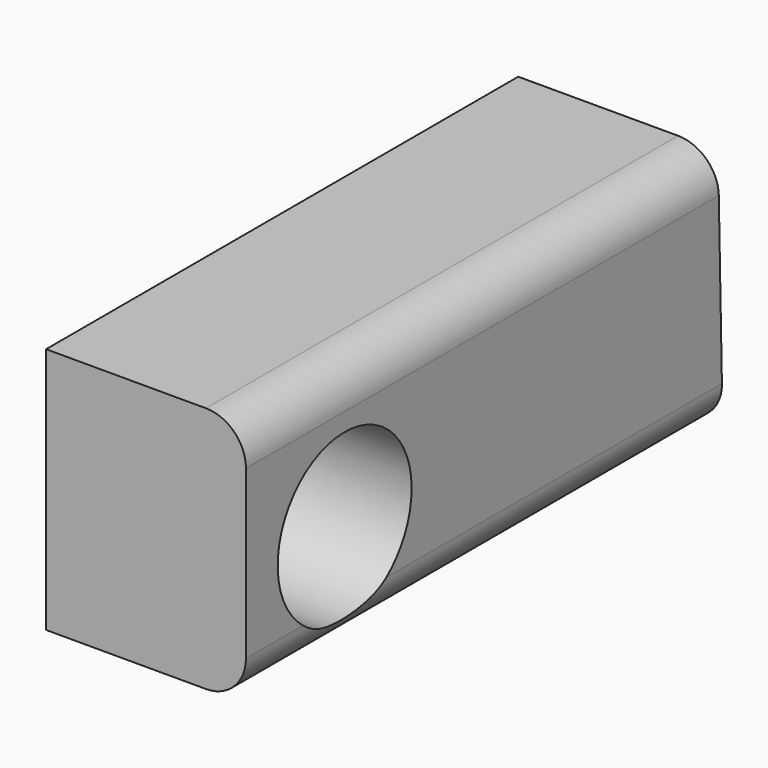
from build123d import *

# Parameters (mm, degrees)
F1_R        = 10.6370455912
F2_DEPTH    = 25.4
F3_T1_DEPTH = 100.398319149
F3_T3_DEPTH = 101.1274702191


# Not quite as in the source:
# - a fillet or chamfer that OpenCascade refuses, or shapes differently, is made with other operations: its cross-section is extruded or revolved along the edge and cut away or added


with BuildPart() as f2:
    # F1 (on face) → F2 (new body)
    with BuildSketch(Plane.YZ):
        Polygon((0, 19.1946215928), (75.7274702191, 19.1946215928), (74.998319149, 50.6070703268), (0, 50.6070703268), align=None)
        with Locations((15.6783070415, 32.5921848416)):
            Circle(F1_R, mode=Mode.SUBTRACT)
    extrude(amount=F2_DEPTH)

    # F3: fillet of radius 5.08 on 2 edges, made by hand

    # F3_s2 → F3_t1 (cut)
    with BuildSketch(Plane.XZ.offset(-87.698319149)):
        with BuildLine():
            ThreePointArc((20.32, 50.6070703268), (23.9121024484, 49.1191727752), (25.4, 45.5270703268))
            Line((25.4, 45.5270703268), (25.4, 50.6070703268))
            Line((25.4, 50.6070703268), (20.32, 50.6070703268))
        make_face()
    extrude(amount=F3_T1_DEPTH, mode=Mode.SUBTRACT)

    # F3_s4 → F3_t3 (cut)
    with BuildSketch(Plane.XZ.offset(-88.4274702191)):
        with BuildLine():
            ThreePointArc((20.32, 19.1946215928), (23.9121024484, 20.6825191443), (25.4, 24.2746215928))
            Line((25.4, 24.2746215928), (25.4, 19.1946215928))
            Line((25.4, 19.1946215928), (20.32, 19.1946215928))
        make_face()
    extrude(amount=F3_T3_DEPTH, mode=Mode.SUBTRACT)


solid = f2.part
